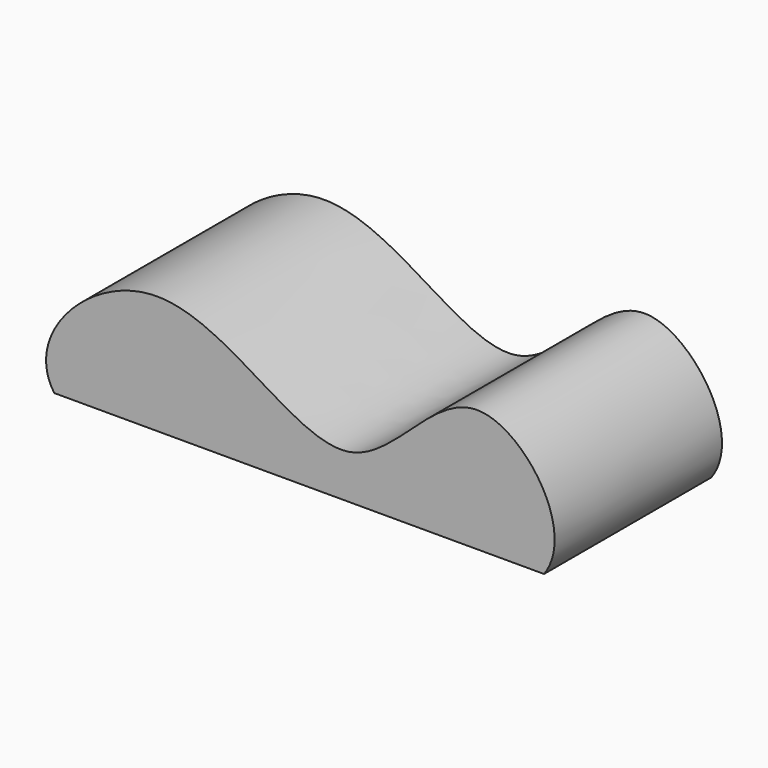
from build123d import *

# Parameters (mm, degrees)
F1_DEPTH = 99.4959305972


with BuildPart() as f1:
    # F0 (on Front) → F1 (new body)
    with BuildSketch(Plane.XZ):
        with BuildLine():
            add(Edge.make_bspline(
                [(-110.9823137522, 0), (-126.0468532321, 21.719385534), (-57.5038619045, 93.268154866), (30.1193231256, -17.739157856), (86.0951259075, 93.5844051862), (137.940946041, 22.1720869346), (121.9706833363, 0)],
                knots=[0, 0, 0, 0, 0.1692301092, 0.3673184606, 0.5367175703, 0.6974891295, 0.6974891295, 0.6974891295, 0.6974891295], degree=3))
            Line((-110.9823137522, 0), (121.9706833363, 0))
        make_face()
    extrude(amount=-F1_DEPTH)


solid = f1.part
